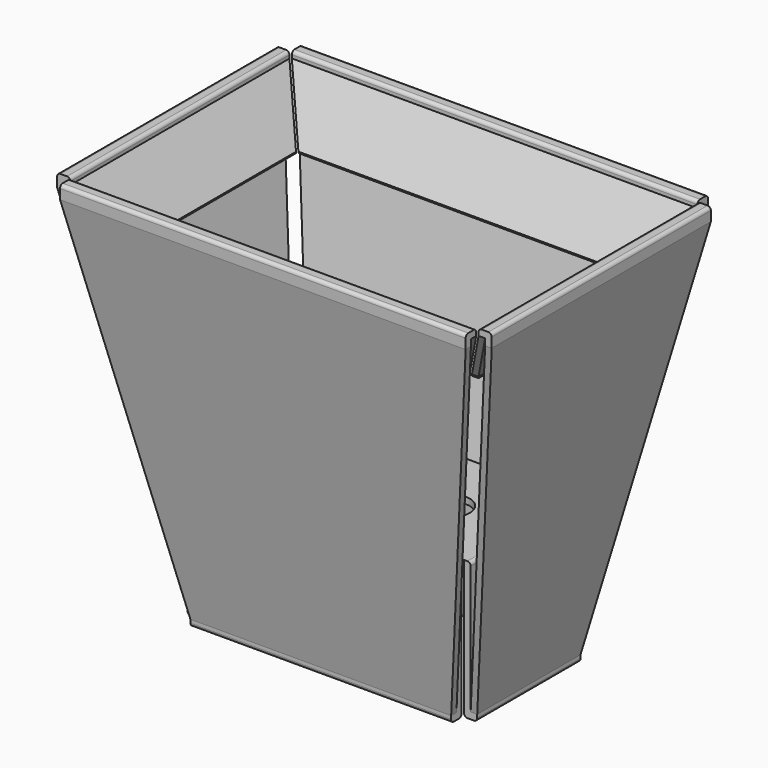
from build123d import *

# Parameters (mm, degrees)
F0_W         = 19.8
F0_H         = 0.5
F0_R         = 1.5
F0_W_2       = 0.5
F0_H_2       = 9.8
F1_DEPTH     = 0.5
F3_W         = 0.5
F3_H         = 9.8
F4_DEPTH     = 1
F3_W_2       = 19.8
F3_H_2       = 0.5
F5_DEPTH     = 0.5
F4_FACE_W    = 19.8
F4_FACE_H    = 0.5
F4_FACE_W_2  = 0.5
F4_FACE_H_2  = 9.8
F11_R        = 0.25
F11_2_R      = 0.25
F11_3_R      = 0.25
F11_4_R      = 0.25
F11_5_R      = 0.25
F2_W         = 30.8
F2_H         = 0.5
F12_DEPTH    = 1
F2_W_2       = 0.5
F2_H_2       = 20.8
F13_DEPTH    = 0.5
F5_FACE_W    = 0.5
F5_FACE_H    = 9.8
F12_FACE_W   = 0.5
F12_FACE_H   = 20.8
F5_FACE_W_2  = 19.8
F5_FACE_H_2  = 0.5
F12_FACE_W_2 = 30.8
F12_FACE_H_2 = 0.5
F19_W        = 0.5
F19_H        = 15.8
F20_DEPTH    = 0.1
F19_W_2      = 25.8
F19_H_2      = 0.5
F13_FACE_W   = 0.5
F13_FACE_H   = 20.8
F20_FACE_W   = 0.5
F20_FACE_H   = 15.8
F13_FACE_W_2 = 30.8
F13_FACE_H_2 = 0.5
F20_FACE_W_2 = 25.8
F20_FACE_H_2 = 0.5
F26_R        = 0.25
F27_R        = 0.25
F28_R        = 0.25


with BuildPart() as f1:
    # F0 (on Top) → F1 (new body)
    with BuildSketch(Plane.XY):
        with Locations((0, 5.25)):
            Rectangle(F0_W, F0_H)
        Polygon((9.9, 5), (-9.9, 5), (-10, 4.9), (-10, -4.9), (-9.9, -5), (9.9, -5), (10, -4.9), (10, 4.9), align=None)
        with Locations((-5, 0)):
            Circle(F0_R, mode=Mode.SUBTRACT)
        with Locations((5, 0)):
            Circle(F0_R, mode=Mode.SUBTRACT)
        with Locations((-10.25, 0)):
            Rectangle(F0_W_2, F0_H_2)
        with Locations((10.25, 0)):
            Rectangle(F0_W_2, F0_H_2)
        with Locations((0, -5.25)):
            Rectangle(F0_W, F0_H)
    extrude(amount=F1_DEPTH)



with BuildPart() as f4:
    # F3 (on face) → F4 (new body)
    with BuildSketch(Plane(origin=(0, 0, 0), x_dir=(1, 0, 0), z_dir=(0, 0, -1))):
        with Locations((10.25, 0)):
            Rectangle(F3_W, F3_H)
    extrude(amount=-F4_DEPTH)


with BuildPart() as f4b:
    # F3 (on face) → F4, piece 2 (new body)
    with BuildSketch(Plane(origin=(0, 0, 0), x_dir=(1, 0, 0), z_dir=(0, 0, -1))):
        with Locations((0, -5.25)):
            Rectangle(F3_W_2, F3_H_2)
    extrude(amount=-F4_DEPTH)


with BuildPart() as f4c:
    # F3 (on face) → F4, piece 3 (new body)
    with BuildSketch(Plane(origin=(0, 0, 0), x_dir=(1, 0, 0), z_dir=(0, 0, -1))):
        with Locations((0, 5.25)):
            Rectangle(F3_W_2, F3_H_2)
    extrude(amount=-F4_DEPTH)


with BuildPart() as f4d:
    # F3 (on face) → F4, piece 4 (new body)
    with BuildSketch(Plane(origin=(0, 0, 0), x_dir=(1, 0, 0), z_dir=(0, 0, -1))):
        with Locations((-10.25, 0)):
            Rectangle(F3_W, F3_H)
    extrude(amount=-F4_DEPTH)


with BuildPart() as f5:
    # F3 (on face) → F5 (new body)
    with BuildSketch(Plane(origin=(0, 0, 0), x_dir=(1, 0, 0), z_dir=(0, 0, -1))):
        with Locations((0, -5.75)):
            Rectangle(F3_W_2, F3_H_2)
    extrude(amount=-F5_DEPTH)


with BuildPart() as f5b:
    # F3 (on face) → F5, piece 2 (new body)
    with BuildSketch(Plane(origin=(0, 0, 0), x_dir=(1, 0, 0), z_dir=(0, 0, -1))):
        with Locations((0, 5.75)):
            Rectangle(F3_W_2, F3_H_2)
    extrude(amount=-F5_DEPTH)


with BuildPart() as f5c:
    # F3 (on face) → F5, piece 3 (new body)
    with BuildSketch(Plane(origin=(0, 0, 0), x_dir=(1, 0, 0), z_dir=(0, 0, -1))):
        with Locations((-10.75, 0)):
            Rectangle(F3_W, F3_H)
    extrude(amount=-F5_DEPTH)


with BuildPart() as f5d:
    # F3 (on face) → F5, piece 4 (new body)
    with BuildSketch(Plane(origin=(0, 0, 0), x_dir=(1, 0, 0), z_dir=(0, 0, -1))):
        with Locations((10.75, 0)):
            Rectangle(F3_W, F3_H)
    extrude(amount=-F5_DEPTH)


with BuildPart() as f4c_1:
    # F6: moved
    add(f4c.part.moved(Location((0, 0, -10))))


with BuildPart() as f5b_1:
    # F6: moved
    add(f5b.part.moved(Location((0, 0, -10))))

    # F11#3
    f11_3_edges = [f5b_1.edges().sort_by_distance(p)[0] for p in [
        (0, -6, -10),
    ]]
    fillet(f11_3_edges, radius=F11_3_R)


with BuildPart() as f5d_1:
    # F6: moved
    add(f5d.part.moved(Location((0, 0, -10))))

    # F11#5
    f11_5_edges = [f5d_1.edges().sort_by_distance(p)[0] for p in [
        (11, 0, -10),
    ]]
    fillet(f11_5_edges, radius=F11_5_R)


with BuildPart() as f4_1:
    # F6: moved
    add(f4.part.moved(Location((0, 0, -10))))


with BuildPart() as f5_1:
    # F6: moved
    add(f5.part.moved(Location((0, 0, -10))))

    # F11#2
    f11_2_edges = [f5_1.edges().sort_by_distance(p)[0] for p in [
        (0, 6, -10),
    ]]
    fillet(f11_2_edges, radius=F11_2_R)


with BuildPart() as f4b_1:
    # F6: moved
    add(f4b.part.moved(Location((0, 0, -10))))


with BuildPart() as f5c_1:
    # F6: moved
    add(f5c.part.moved(Location((0, 0, -10))))

    # F11#4
    f11_4_edges = [f5c_1.edges().sort_by_distance(p)[0] for p in [
        (-11, 0, -10),
    ]]
    fillet(f11_4_edges, radius=F11_4_R)


with BuildPart() as f4d_1:
    # F6: moved
    add(f4d.part.moved(Location((0, 0, -10))))


with BuildPart() as f1_1:
    add(f1.part)

    add(f4c_1.part)  # F7 merges F4c
    # F4_face (on face) → F7 section 0
    with BuildSketch(Plane(origin=(0, -5.25, -9), x_dir=(1, 0, 0), z_dir=(0, 0, 1))):
        Rectangle(F4_FACE_W, F4_FACE_H)
    # F0 (on Top) → F7 section 1
    with BuildSketch(Plane.XY):
        with Locations((0, -5.25)):
            Rectangle(F0_W, F0_H)
    loft()


    add(f4_1.part)  # F8 merges F4
    # F0 (on Top) → F8 section 0
    with BuildSketch(Plane.XY):
        with Locations((10.25, 0)):
            Rectangle(F0_W_2, F0_H_2)
    # F4_face (on face) → F8 section 1
    with BuildSketch(Plane(origin=(0, -5.25, -9), x_dir=(1, 0, 0), z_dir=(0, 0, 1))):
        with Locations((10.25, 5.25)):
            Rectangle(F4_FACE_W_2, F4_FACE_H_2)
    loft()


    add(f4b_1.part)  # F9 merges F4b
    # F0 (on Top) → F9 section 0
    with BuildSketch(Plane.XY):
        with Locations((0, 5.25)):
            Rectangle(F0_W, F0_H)
    # F4_face (on face) → F9 section 1
    with BuildSketch(Plane(origin=(0, -5.25, -9), x_dir=(1, 0, 0), z_dir=(0, 0, 1))):
        with Locations((0, 10.5)):
            Rectangle(F4_FACE_W, F4_FACE_H)
    loft()


    add(f4d_1.part)  # F10 merges F4d
    # F0 (on Top) → F10 section 0
    with BuildSketch(Plane.XY):
        with Locations((-10.25, 0)):
            Rectangle(F0_W_2, F0_H_2)
    # F4_face (on face) → F10 section 1
    with BuildSketch(Plane(origin=(0, -5.25, -9), x_dir=(1, 0, 0), z_dir=(0, 0, 1))):
        with Locations((-10.25, 5.25)):
            Rectangle(F4_FACE_W_2, F4_FACE_H_2)
    loft()

    # F11
    f11_edges = [f1_1.edges().sort_by_distance(p)[0] for p in [
        (10.5, 0, 0.5),
        (0, -5.5, 0.5),
        (0, 5.5, 0.5),
        (-10.5, 0, 0.5),
        (-10, 0, -10),
        (0, 5, -10),
        (10, 0, -10),
        (0, -5, -10),
    ]]
    fillet(f11_edges, radius=F11_R)


    add(f5c_1.part)  # F15 merges F5c


with BuildPart() as f12:
    # F2 (on Top) → F12 (new body)
    with BuildSketch(Plane.XY):
        with Locations((0, 11.25)):
            Rectangle(F2_W, F2_H)
    extrude(amount=-F12_DEPTH)


with BuildPart() as f12b:
    # F2 (on Top) → F12, piece 2 (new body)
    with BuildSketch(Plane.XY):
        with Locations((-16.25, 0)):
            Rectangle(F2_W_2, F2_H_2)
    extrude(amount=-F12_DEPTH)


with BuildPart() as f12c:
    # F2 (on Top) → F12, piece 3 (new body)
    with BuildSketch(Plane.XY):
        with Locations((0, -11.25)):
            Rectangle(F2_W, F2_H)
    extrude(amount=-F12_DEPTH)


with BuildPart() as f12d:
    # F2 (on Top) → F12, piece 4 (new body)
    with BuildSketch(Plane.XY):
        with Locations((16.25, 0)):
            Rectangle(F2_W_2, F2_H_2)
    extrude(amount=-F12_DEPTH)


with BuildPart() as f13:
    # F2 (on Top) → F13 (new body)
    with BuildSketch(Plane.XY):
        with Locations((-15.75, 0)):
            Rectangle(F2_W_2, F2_H_2)
    extrude(amount=-F13_DEPTH)


with BuildPart() as f13b:
    # F2 (on Top) → F13, piece 2 (new body)
    with BuildSketch(Plane.XY):
        with Locations((0, 10.75)):
            Rectangle(F2_W, F2_H)
    extrude(amount=-F13_DEPTH)


with BuildPart() as f13c:
    # F2 (on Top) → F13, piece 3 (new body)
    with BuildSketch(Plane.XY):
        with Locations((15.75, 0)):
            Rectangle(F2_W_2, F2_H_2)
    extrude(amount=-F13_DEPTH)


with BuildPart() as f13d:
    # F2 (on Top) → F13, piece 4 (new body)
    with BuildSketch(Plane.XY):
        with Locations((0, -10.75)):
            Rectangle(F2_W, F2_H)
    extrude(amount=-F13_DEPTH)


with BuildPart() as f13b_1:
    # F14: moved
    add(f13b.part.moved(Location((0, 0, 20))))


with BuildPart() as f12_1:
    # F14: moved
    add(f12.part.moved(Location((0, 0, 20))))


with BuildPart() as f12b_1:
    # F14: moved
    add(f12b.part.moved(Location((0, 0, 20))))


with BuildPart() as f13_1:
    # F14: moved
    add(f13.part.moved(Location((0, 0, 20))))


with BuildPart() as f13d_1:
    # F14: moved
    add(f13d.part.moved(Location((0, 0, 20))))


with BuildPart() as f12c_1:
    # F14: moved
    add(f12c.part.moved(Location((0, 0, 20))))


with BuildPart() as f13c_1:
    # F14: moved
    add(f13c.part.moved(Location((0, 0, 20))))


with BuildPart() as f12d_1:
    # F14: moved
    add(f12d.part.moved(Location((0, 0, 20))))


with BuildPart() as f1_2:
    add(f1_1.part)

    add(f12b_1.part)  # F15 merges F12b
    # F5_face (on face) → F15 section 0
    with BuildSketch(Plane(origin=(-10.75, 0, -9.5), x_dir=(1, 0, 0), z_dir=(0, 0, 1))):
        Rectangle(F5_FACE_W, F5_FACE_H)
    # F12_face (on face) → F15 section 1
    with BuildSketch(Plane(origin=(-16.25, 0, 19), x_dir=(1, 0, 0), z_dir=(0, 0, -1))):
        Rectangle(F12_FACE_W, F12_FACE_H)
    loft()


    add(f5b_1.part)  # F16 merges F5b

    add(f12c_1.part)  # F16 merges F12c
    # F5_face (on face) → F16 section 0
    with BuildSketch(Plane(origin=(-10.75, 0, -9.5), x_dir=(1, 0, 0), z_dir=(0, 0, 1))):
        with Locations((10.75, -5.75)):
            Rectangle(F5_FACE_W_2, F5_FACE_H_2)
    # F12_face (on face) → F16 section 1
    with BuildSketch(Plane(origin=(-16.25, 0, 19), x_dir=(1, 0, 0), z_dir=(0, 0, -1))):
        with Locations((16.25, 11.25)):
            Rectangle(F12_FACE_W_2, F12_FACE_H_2)
    loft()


    add(f5d_1.part)  # F17 merges F5d

    add(f12d_1.part)  # F17 merges F12d
    # F5_face (on face) → F17 section 0
    with BuildSketch(Plane(origin=(-10.75, 0, -9.5), x_dir=(1, 0, 0), z_dir=(0, 0, 1))):
        with Locations((21.5, 0)):
            Rectangle(F5_FACE_W, F5_FACE_H)
    # F12_face (on face) → F17 section 1
    with BuildSketch(Plane(origin=(-16.25, 0, 19), x_dir=(1, 0, 0), z_dir=(0, 0, -1))):
        with Locations((32.5, 0)):
            Rectangle(F12_FACE_W, F12_FACE_H)
    loft()


    add(f5_1.part)  # F18 merges F5

    add(f12_1.part)  # F18 merges F12
    # F5_face (on face) → F18 section 0
    with BuildSketch(Plane(origin=(-10.75, 0, -9.5), x_dir=(1, 0, 0), z_dir=(0, 0, 1))):
        with Locations((10.75, 5.75)):
            Rectangle(F5_FACE_W_2, F5_FACE_H_2)
    # F12_face (on face) → F18 section 1
    with BuildSketch(Plane(origin=(-16.25, 0, 19), x_dir=(1, 0, 0), z_dir=(0, 0, -1))):
        with Locations((16.25, -11.25)):
            Rectangle(F12_FACE_W_2, F12_FACE_H_2)
    loft()


    add(f13_1.part)  # F22 merges F13


with BuildPart() as f20:
    # F19 (on Top) → F20 (new body)
    with BuildSketch(Plane.XY):
        with Locations((-13.25, 0)):
            Rectangle(F19_W, F19_H)
    extrude(amount=F20_DEPTH)


with BuildPart() as f20b:
    # F19 (on Top) → F20, piece 2 (new body)
    with BuildSketch(Plane.XY):
        with Locations((0, -8.25)):
            Rectangle(F19_W_2, F19_H_2)
    extrude(amount=F20_DEPTH)


with BuildPart() as f20c:
    # F19 (on Top) → F20, piece 3 (new body)
    with BuildSketch(Plane.XY):
        with Locations((13.25, 0)):
            Rectangle(F19_W, F19_H)
    extrude(amount=F20_DEPTH)


with BuildPart() as f20d:
    # F19 (on Top) → F20, piece 4 (new body)
    with BuildSketch(Plane.XY):
        with Locations((0, 8.25)):
            Rectangle(F19_W_2, F19_H_2)
    extrude(amount=F20_DEPTH)


with BuildPart() as f20b_1:
    # F21: moved
    add(f20b.part.moved(Location((0, 0, 15))))


with BuildPart() as f20d_1:
    # F21: moved
    add(f20d.part.moved(Location((0, 0, 15))))


with BuildPart() as f20c_1:
    # F21: moved
    add(f20c.part.moved(Location((0, 0, 15))))


with BuildPart() as f20_1:
    # F21: moved
    add(f20.part.moved(Location((0, 0, 15))))


with BuildPart() as f1_3:
    add(f1_2.part)

    add(f20_1.part)  # F22 merges F20
    # F13_face (on face) → F22 section 0
    with BuildSketch(Plane(origin=(-15.75, 0, 19.5), x_dir=(1, 0, 0), z_dir=(0, 0, -1))):
        Rectangle(F13_FACE_W, F13_FACE_H)
    # F20_face (on face) → F22 section 1
    with BuildSketch(Plane(origin=(-13.25, 0, 15.1), x_dir=(1, 0, 0), z_dir=(0, 0, 1))):
        Rectangle(F20_FACE_W, F20_FACE_H)
    loft()


    add(f13b_1.part)  # F23 merges F13b

    add(f20d_1.part)  # F23 merges F20d
    # F13_face (on face) → F23 section 0
    with BuildSketch(Plane(origin=(-15.75, 0, 19.5), x_dir=(1, 0, 0), z_dir=(0, 0, -1))):
        with Locations((15.75, -10.75)):
            Rectangle(F13_FACE_W_2, F13_FACE_H_2)
    # F20_face (on face) → F23 section 1
    with BuildSketch(Plane(origin=(-13.25, 0, 15.1), x_dir=(1, 0, 0), z_dir=(0, 0, 1))):
        with Locations((13.25, 8.25)):
            Rectangle(F20_FACE_W_2, F20_FACE_H_2)
    loft()


    add(f13d_1.part)  # F24 merges F13d

    add(f20b_1.part)  # F24 merges F20b
    # F20_face (on face) → F24 section 0
    with BuildSketch(Plane(origin=(-13.25, 0, 15.1), x_dir=(1, 0, 0), z_dir=(0, 0, 1))):
        with Locations((13.25, -8.25)):
            Rectangle(F20_FACE_W_2, F20_FACE_H_2)
    # F13_face (on face) → F24 section 1
    with BuildSketch(Plane(origin=(-15.75, 0, 19.5), x_dir=(1, 0, 0), z_dir=(0, 0, -1))):
        with Locations((15.75, 10.75)):
            Rectangle(F13_FACE_W_2, F13_FACE_H_2)
    loft()


    add(f13c_1.part)  # F25 merges F13c

    add(f20c_1.part)  # F25 merges F20c
    # F13_face (on face) → F25 section 0
    with BuildSketch(Plane(origin=(-15.75, 0, 19.5), x_dir=(1, 0, 0), z_dir=(0, 0, -1))):
        with Locations((31.5, 0)):
            Rectangle(F13_FACE_W, F13_FACE_H)
    # F20_face (on face) → F25 section 1
    with BuildSketch(Plane(origin=(-13.25, 0, 15.1), x_dir=(1, 0, 0), z_dir=(0, 0, 1))):
        with Locations((26.5, 0)):
            Rectangle(F20_FACE_W, F20_FACE_H)
    loft()

    # F26
    f26_edges = [f1_3.edges().sort_by_distance(p)[0] for p in [
        (-15.5, 0, 20),
    ]]
    fillet(f26_edges, radius=F26_R)

    # F27
    f27_edges = [f1_3.edges().sort_by_distance(p)[0] for p in [
        (0, 10.5, 20),
        (15.5, 0, 20),
        (0, -10.5, 20),
    ]]
    fillet(f27_edges, radius=F27_R)

    # F28
    f28_edges = [f1_3.edges().sort_by_distance(p)[0] for p in [
        (16.5, 0, 20),
        (0, -11.5, 20),
        (0, 11.5, 20),
        (-16.5, 0, 20),
    ]]
    fillet(f28_edges, radius=F28_R)


solid = f1_3.part
